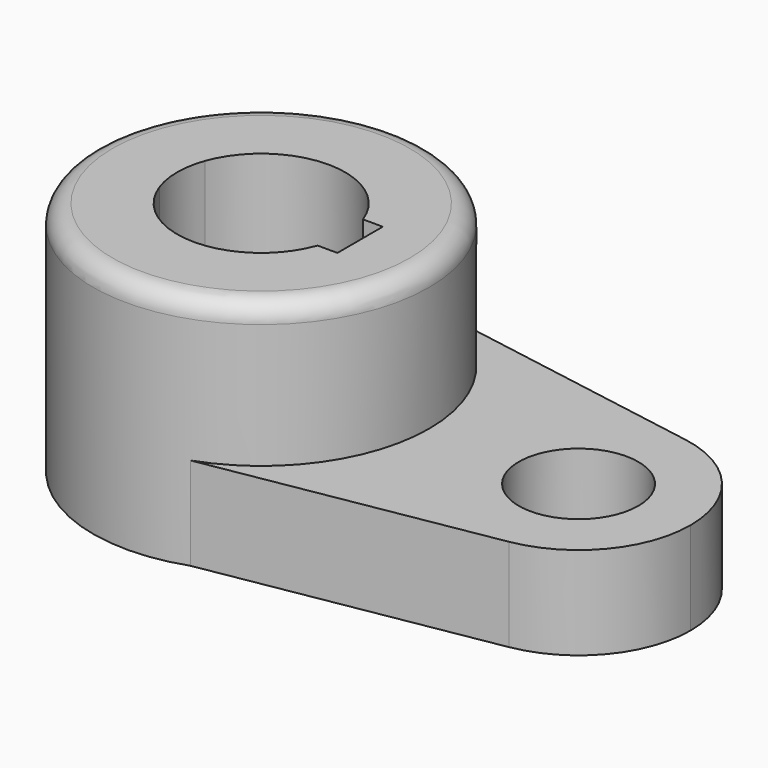
from build123d import *

# Parameters (mm, degrees)
F0_R     = 28.575
F1_DEPTH = 40.2336
F2_R     = 10.16
F3_DEPTH = 15.7734
F4_DEPTH = 25.4
F5_R     = 3.302


with BuildPart() as f1:
    # F0 (on Top) → F1 (new body)
    with BuildSketch(Plane.XY):
        Circle(F0_R)
        with BuildLine():
            ThreePointArc((-13.4477648793, -4.826), (-14.2875, 0), (-13.4477648793, 4.826))
            ThreePointArc((-13.4477648793, 4.826), (0, 14.2875), (13.4477648793, 4.826))
            Line((13.4477648793, 4.826), (16.8290351207, 4.826))
            Line((16.8290351207, 4.826), (16.8290351207, -4.826))
            Line((16.8290351207, -4.826), (13.4477648793, -4.826))
            ThreePointArc((13.4477648793, -4.826), (0, -14.2875), (-13.4477648793, -4.826))
        make_face(mode=Mode.SUBTRACT)
    extrude(amount=F1_DEPTH)

    # F2 (on Top) → F3 (join)
    with BuildSketch(Plane.XY):
        with BuildLine():
            ThreePointArc((57.1919272622, -18.7764181619), (34.925, 0), (57.1919272622, 18.7764181619))
            Line((57.1919272622, 18.7764181619), (9.5121844836, 26.9452959039))
            ThreePointArc((9.5121844836, 26.9452959039), (23.3274655355, 16.5033322905), (28.575, 0))
            ThreePointArc((28.575, 0), (23.3274655355, -16.5033322905), (9.5121844836, -26.9452959039))
            Line((9.5121844836, -26.9452959039), (57.1919272622, -18.7764181619))
        make_face()
        with BuildLine():
            ThreePointArc((57.1919272622, -18.7764181619), (68.5383952831, -12.2804730295), (73.025, 0))
            ThreePointArc((73.025, 0), (68.5383952831, 12.2804730295), (57.1919272622, 18.7764181619))
            ThreePointArc((57.1919272622, 18.7764181619), (34.925, 0), (57.1919272622, -18.7764181619))
        make_face()
        with Locations((53.975, 0)):
            Circle(F2_R, mode=Mode.SUBTRACT)
    extrude(amount=F3_DEPTH)

    # F0 (on Top) → F4 (join)
    with BuildSketch(Plane.XY):
        Circle(F0_R)
        with BuildLine():
            ThreePointArc((-13.4477648793, -4.826), (-14.2875, 0), (-13.4477648793, 4.826))
            ThreePointArc((-13.4477648793, 4.826), (0, 14.2875), (13.4477648793, 4.826))
            Line((13.4477648793, 4.826), (16.8290351207, 4.826))
            Line((16.8290351207, 4.826), (16.8290351207, -4.826))
            Line((16.8290351207, -4.826), (13.4477648793, -4.826))
            ThreePointArc((13.4477648793, -4.826), (0, -14.2875), (-13.4477648793, -4.826))
        make_face(mode=Mode.SUBTRACT)
    extrude(amount=F4_DEPTH)

    # F5
    f5_edges = [f1.edges().sort_by_distance(p)[0] for p in [
        (-28.575, 0, 40.2336),
    ]]
    fillet(f5_edges, radius=F5_R)


solid = f1.part
